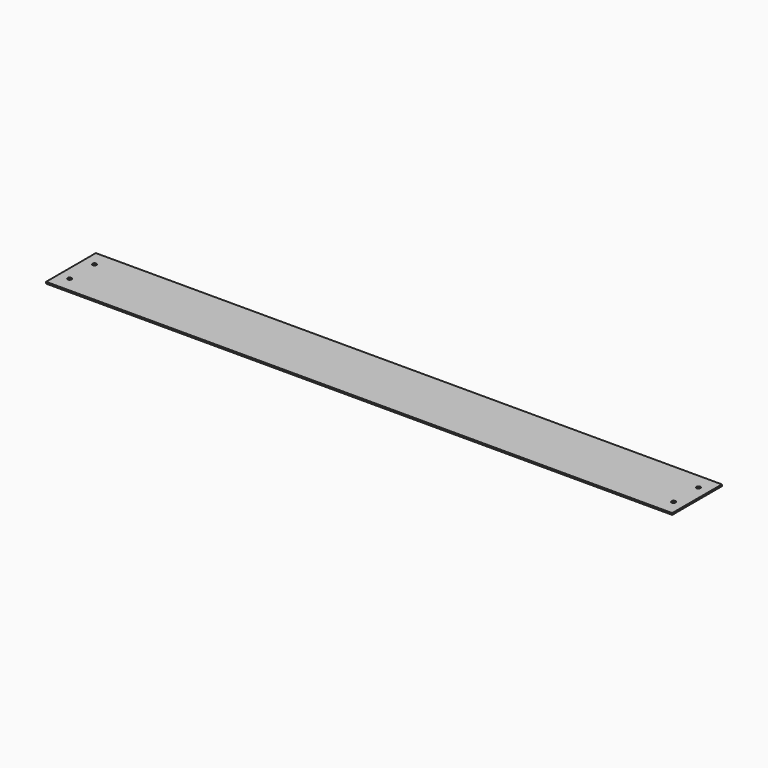
from build123d import *

# Parameters (mm, degrees)
F0_W     = 355.6
F0_H     = 9.525
F1_DEPTH = 1790.7
F3_DEPTH = 25.4


# Not quite as in the source:
# - a fillet or chamfer that OpenCascade refuses, or shapes differently, is made with other operations: its cross-section is extruded or revolved along the edge and cut away or added


with BuildPart() as f1:
    # F0 (on Right) → F1 (new body, symmetric)
    with BuildSketch(Plane.YZ):
        Rectangle(F0_W, F0_H)
    extrude(amount=F1_DEPTH, both=True)

    # F2 (on face) → F3 (cut)
    with BuildSketch(Plane.XY.offset(4.7625)):
        with BuildLine():
            Line((-1727.2, 88.9), (-1735.5439, 88.9))
            ThreePointArc((-1735.5439, 88.9), (-1733.1000282715, 82.9999717285), (-1727.2, 80.5561))
            Line((-1727.2, 80.5561), (-1727.2, 88.9))
        make_face()
        with BuildLine():
            Line((-1718.8561, 88.9), (-1727.2, 88.9))
            Line((-1727.2, 88.9), (-1727.2, 80.5561))
            ThreePointArc((-1727.2, 80.5561), (-1721.2999717285, 82.9999717285), (-1718.8561, 88.9))
        make_face()
        with BuildLine():
            ThreePointArc((-1718.8561, 88.9), (-1721.2999717285, 94.8000282715), (-1727.2, 97.2439))
            Line((-1727.2, 97.2439), (-1727.2, 88.9))
            Line((-1727.2, 88.9), (-1718.8561, 88.9))
        make_face()
        with BuildLine():
            ThreePointArc((-1727.2, 97.2439), (-1733.1000282715, 94.8000282715), (-1735.5439, 88.9))
            Line((-1735.5439, 88.9), (-1727.2, 88.9))
            Line((-1727.2, 88.9), (-1727.2, 97.2439))
        make_face()
        with BuildLine():
            ThreePointArc((1735.5439, -88.9), (1733.1000282715, -82.9999717285), (1727.2, -80.5561))
            Line((1727.2, -80.5561), (1727.2, -88.9))
            Line((1727.2, -88.9), (1735.5439, -88.9))
        make_face()
        with BuildLine():
            ThreePointArc((1727.2, -80.5561), (1721.2999717285, -82.9999717285), (1718.8561, -88.9))
            Line((1718.8561, -88.9), (1727.2, -88.9))
            Line((1727.2, -88.9), (1727.2, -80.5561))
        make_face()
        with BuildLine():
            Line((1735.5439, -88.9), (1727.2, -88.9))
            Line((1727.2, -88.9), (1727.2, -97.2439))
            ThreePointArc((1727.2, -97.2439), (1733.1000282715, -94.8000282715), (1735.5439, -88.9))
        make_face()
        with BuildLine():
            Line((1727.2, -88.9), (1718.8561, -88.9))
            ThreePointArc((1718.8561, -88.9), (1721.2999717285, -94.8000282715), (1727.2, -97.2439))
            Line((1727.2, -97.2439), (1727.2, -88.9))
        make_face()
        with BuildLine():
            Line((1727.2, 88.9), (1718.8561, 88.9))
            ThreePointArc((1718.8561, 88.9), (1721.2999717285, 82.9999717285), (1727.2, 80.5561))
            Line((1727.2, 80.5561), (1727.2, 88.9))
        make_face()
        with BuildLine():
            Line((1727.2, 88.9), (1727.2, 97.2439))
            ThreePointArc((1727.2, 97.2439), (1721.2999717285, 94.8000282715), (1718.8561, 88.9))
            Line((1718.8561, 88.9), (1727.2, 88.9))
        make_face()
        with BuildLine():
            ThreePointArc((1735.5439, 88.9), (1733.1000282715, 94.8000282715), (1727.2, 97.2439))
            Line((1727.2, 97.2439), (1727.2, 88.9))
            Line((1727.2, 88.9), (1735.5439, 88.9))
        make_face()
        with BuildLine():
            Line((1735.5439, 88.9), (1727.2, 88.9))
            Line((1727.2, 88.9), (1727.2, 80.5561))
            ThreePointArc((1727.2, 80.5561), (1733.1000282715, 82.9999717285), (1735.5439, 88.9))
        make_face()
        with BuildLine():
            ThreePointArc((-1727.2, -80.5561), (-1733.1000282715, -82.9999717285), (-1735.5439, -88.9))
            Line((-1735.5439, -88.9), (-1727.2, -88.9))
            Line((-1727.2, -88.9), (-1727.2, -80.5561))
        make_face()
        with BuildLine():
            Line((-1727.2, -80.5561), (-1727.2, -88.9))
            Line((-1727.2, -88.9), (-1718.8561, -88.9))
            ThreePointArc((-1718.8561, -88.9), (-1721.2999717285, -82.9999717285), (-1727.2, -80.5561))
        make_face()
        with BuildLine():
            Line((-1718.8561, -88.9), (-1727.2, -88.9))
            Line((-1727.2, -88.9), (-1727.2, -97.2439))
            ThreePointArc((-1727.2, -97.2439), (-1721.2999717285, -94.8000282715), (-1718.8561, -88.9))
        make_face()
        with BuildLine():
            Line((-1727.2, -88.9), (-1735.5439, -88.9))
            ThreePointArc((-1735.5439, -88.9), (-1733.1000282715, -94.8000282715), (-1727.2, -97.2439))
            Line((-1727.2, -97.2439), (-1727.2, -88.9))
        make_face()
    extrude(amount=-F3_DEPTH, mode=Mode.SUBTRACT)

    # F4: chamfer of 12.7 x 11.9060876876 on 4 edges, made by hand

    # F4_s1 → F4_t2 (revolve, cut)
    with BuildSketch(Plane.XZ.offset(88.9)):
        Polygon((-1747.4499876876, -4.7625), (-1735.5439, 7.9375), (-1735.5439, -4.7625), align=None)
    revolve(axis=Axis((-1727.2, -88.9, -4.7625), (0, 0, 1)), mode=Mode.SUBTRACT)

    # F4_s3 → F4_t4 (revolve, cut)
    with BuildSketch(Plane.YZ.offset(-1727.2)):
        Polygon((109.1499876876, -4.7625), (97.2439, 7.9375), (97.2439, -4.7625), align=None)
    revolve(axis=Axis((-1727.2, 88.9, -4.7625), (0, 0, 1)), mode=Mode.SUBTRACT)

    # F4_s5 → F4_t6 (revolve, cut)
    with BuildSketch(Plane.YZ.offset(1727.2)):
        Polygon((68.6500123124, -4.7625), (80.5561, 7.9375), (80.5561, -4.7625), align=None)
    revolve(axis=Axis((1727.2, 88.9, -4.7625), (0, 0, 1)), mode=Mode.SUBTRACT)

    # F4_s7 → F4_t8 (revolve, cut)
    with BuildSketch(Plane.XZ.offset(88.9)):
        Polygon((1706.9500123124, -4.7625), (1718.8561, 7.9375), (1718.8561, -4.7625), align=None)
    revolve(axis=Axis((1727.2, -88.9, -4.7625), (0, 0, 1)), mode=Mode.SUBTRACT)


solid = f1.part
